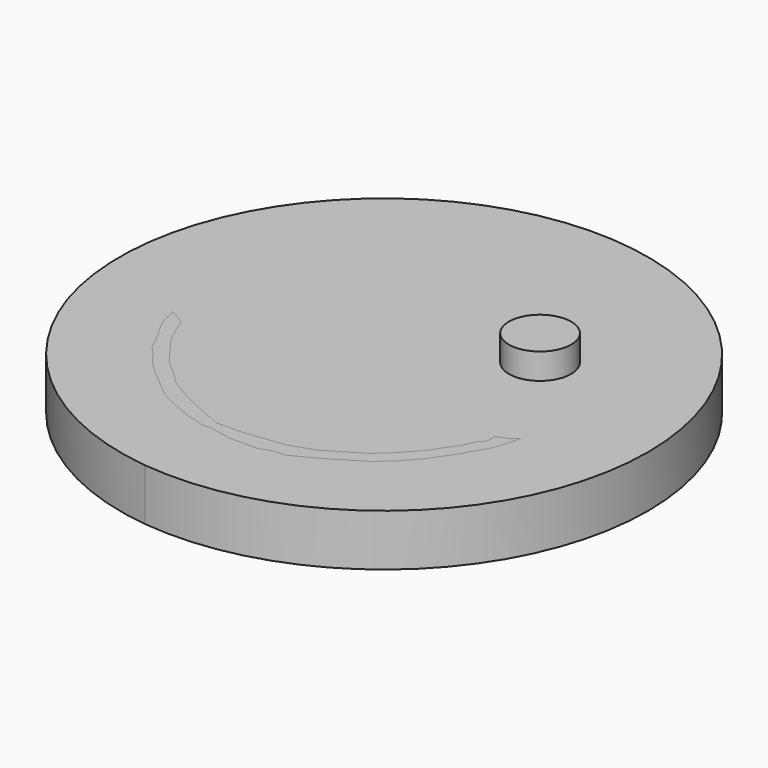
from build123d import *

# Parameters (mm, degrees)
F2_DEPTH  = 10
F3_R      = 6.0161074482
F4_DEPTH  = 5
F9_DEPTH  = 10
F10_DEPTH = 10


# Not quite as in the source:
# - a feature names something its author has since deleted; it is built from what else it names
# - the program builds the solid bodies; features that only make, move or delete a surface that nothing else refers to are left out


with BuildPart() as f2:
    # F1 (on face) → F2 (new body)
    with BuildSketch(Plane.XY):
        with BuildLine():
            ThreePointArc((54.2036075933, -22.7648094296), (-4.7674624295, 27.6592306141), (-45.4207321783, -38.4277013217))
            ThreePointArc((-45.4207321783, -38.4277013217), (-29.0095050887, -62.25377047), (-2.3575475804, -73.5091294881))
            ThreePointArc((-2.3575475804, -73.5091294881), (37.2467444782, -60.7587243792), (54.2036075933, -22.7648094296))
        make_face()
    extrude(amount=F2_DEPTH)

    # F3 (on face) → F4 (join)
    with BuildSketch(Plane.XY.offset(10)):
        with Locations((23.184536978, -10.0657522977)):
            Circle(F3_R)
    extrude(amount=F4_DEPTH)


with BuildPart() as f9:
    # F7 (on face) → F9 (new body, through all)
    with BuildSketch(Plane.XY.offset(10)):
        Polygon((-27.4368692189, -33.4604494274), (-30.4171405733, -31.6883958876), (-29.7727547586, -34.5075726509), (-29.0478244424, -36.3601744175), (-27.8396084905, -38.3738689125), (-26.4702923596, -40.9514009953), (-25.7453620434, -42.6429063082), (-24.2149531841, -44.2538633943), (-22.5234478712, -46.5897507966), (-20.2681086957, -48.7645454705), (-17.5294801593, -51.0198846459), (-14.4686615095, -53.5974167287), (-11.0856518149, -55.2889220417), (-7.0582586341, -56.8998791277), (-3.9168912917, -57.7859058976), (-1.9031949341, -57.7859058976), (1.8020068528, -58.5913844407), (5.6683043949, -58.5913844407), (7.3598097079, -58.5913844407), (10.0178886205, -57.7053576708), (11.9510376826, -57.7053576708), (13.8036385179, -56.8193309009), (16.058979556, -55.6111112237), (17.7504848689, -54.7250844538), (20.4085633159, -53.1141273677), (23.5499292612, -51.1809810996), (26.3691060245, -48.6839972436), (29.1882790625, -45.542627573), (32.1685522795, -41.1930456758), (34.9877253175, -36.2796261907), (35.712659359, -33.9437350631), (36.518137902, -31.1245620251), (35.1488217711, -32.332777977), (32.9740308225, -33.2188047469), (32.9740308225, -35.0714065135), (31.8463593721, -36.2796261907), (30.9603344649, -38.3738689125), (29.3493773788, -40.7097563148), (28.0606094748, -42.8040027618), (26.2080114335, -44.8982454836), (24.1137649864, -47.1535846591), (21.5362329036, -49.4089275599), (18.0726759136, -51.5031702816), (14.7702135146, -53.4363202751), (9.8567930982, -55.0472773612), (2.0436504856, -55.933304131), (-2.628125716, -55.933304131), (-6.4944233745, -54.3223470449), (-11.9716776535, -51.7448149621), (-15.5963320285, -49.4894757867), (-17.6905766129, -47.3952293396), (-20.5902997404, -44.8982454836), (-23.0067353696, -41.6763313115), (-24.939885363, -39.0182510018), (-26.3091977686, -36.1990779638), align=None)
    extrude(amount=-F9_DEPTH)


with BuildPart() as f10:
    # F10 (new, through all): a face of the model
    f10_faces = [f9.part.faces().sort_by_distance(p)[0] for p in [
        (-4.8395499913, -55.7956867711, 10),
    ]]
    extrude(f10_faces, amount=-F10_DEPTH)


solid = Compound([f2.part, f9.part, f10.part])
